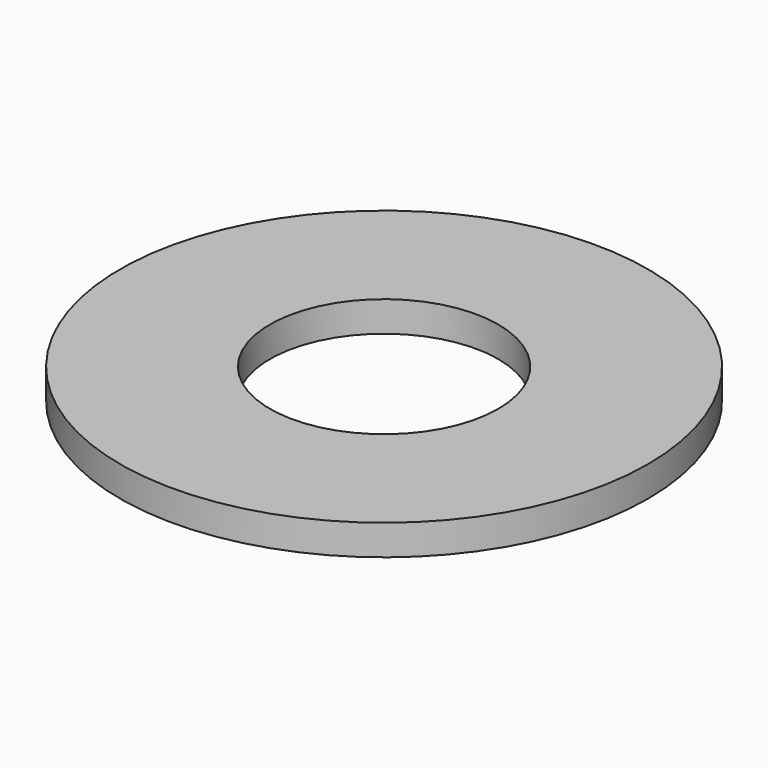
from build123d import *

# Parameters (mm, degrees)
F0_R     = 26
F0_R_2   = 11.25
F1_DEPTH = 3


# Not quite as in the source:
# - a feature names something its author has since deleted; it is built from what else it names


with BuildPart() as f1:
    # F0 (on Top) → F1 (new body)
    with BuildSketch(Plane.XY):
        Circle(F0_R)
        Circle(F0_R_2, mode=Mode.SUBTRACT)
    extrude(amount=-F1_DEPTH)


solid = f1.part
